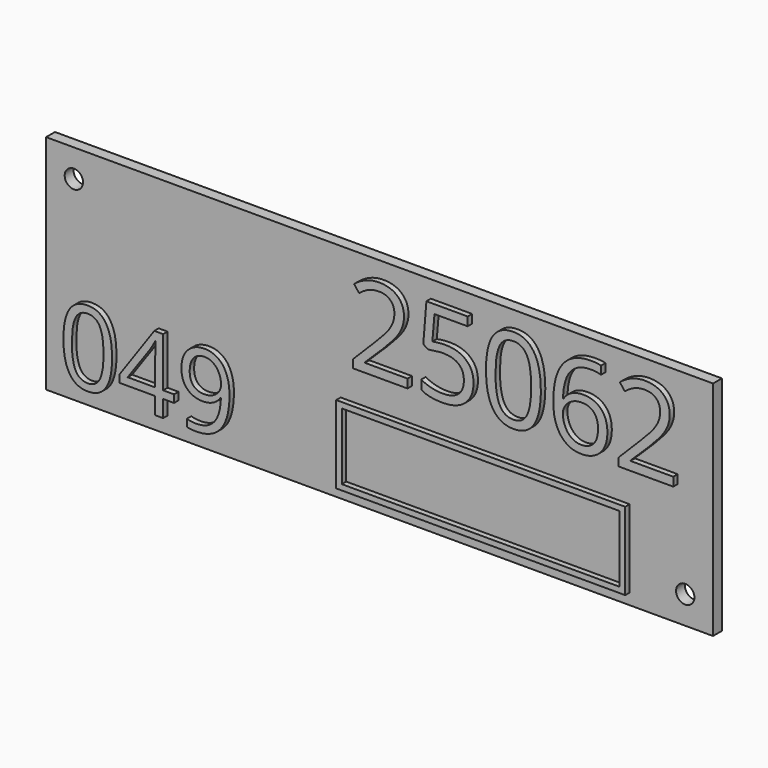
from build123d import *

# Parameters (mm, degrees)
F0_W         = 120
F0_H         = 40
F1_DEPTH     = 2
F3_D         = 3.3
F4_TEXT_SIZE = 20.9070615778
F5_DEPTH     = 1
F6_TEXT_SIZE = 18.5356140827
F7_DEPTH     = 1
F8_W         = 52
F8_H         = 14
F8_W_2       = 49.99999962
F8_H_2       = 11.99999962
F9_DEPTH     = 1


# Not quite as in the source:
# - Text() gives the source's letters only with a copy of the font that has no kerning and outlines rounded to 1/6400 em; it was checked with that copy


with BuildPart() as f1:
    # F0 (on Front) → F1 (new body)
    with BuildSketch(Plane.XZ):
        Rectangle(F0_W, F0_H)
    extrude(amount=F1_DEPTH)

    # F3 (through all)
    with Locations(Plane.XZ.offset(2)):
        with Locations((-55, 15), (55, -15)):
            Hole(F3_D / 2)

    # F4 (on face) → F5 (join)
    with BuildSketch(Plane.XZ.offset(2)):
        with Locations((-5, 2)):
            Text('25062', F4_TEXT_SIZE, font='Open Sans', text_align=(TextAlign.LEFT, TextAlign.BOTTOM))
    extrude(amount=F5_DEPTH)

    # F6 (on face) → F7 (join)
    with BuildSketch(Plane.XZ.offset(2)):
        with Locations((-57, -17)):
            Text('049', F6_TEXT_SIZE, font='Open Sans', text_align=(TextAlign.LEFT, TextAlign.BOTTOM))
    extrude(amount=F7_DEPTH)

    # F8 (on face) → F9 (join)
    with BuildSketch(Plane.XZ.offset(2)):
        with Locations((19, -11)):
            Rectangle(F8_W, F8_H)
        with Locations((19, -11)):
            Rectangle(F8_W_2, F8_H_2, mode=Mode.SUBTRACT)
    extrude(amount=F9_DEPTH)


solid = f1.part
